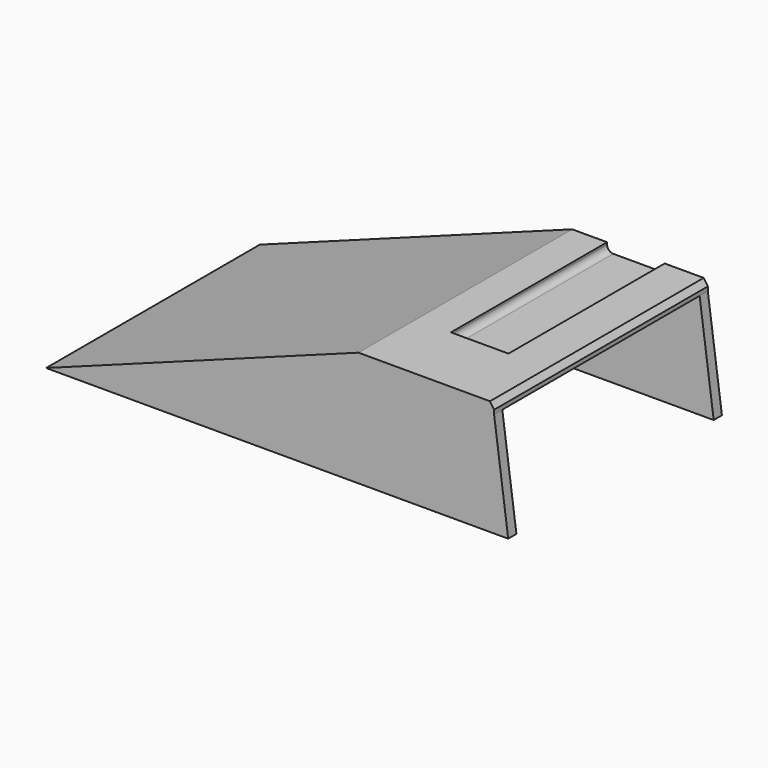
from build123d import *

# Parameters (mm, degrees)
F1_DEPTH      = 6.5
F2_R          = 6
F4_DEPTH      = 0.5
F6_DEPTH      = 3
F6_DEPTH_BACK = 25
F7_SIZE2      = 0.3
F7_SIZE       = 0.2
F8_R          = 0.3


# Not quite as in the source:
# - a pattern or mirror of a feature is missing from the dataset's text; its kind, count and spacing are read off the source's solid


with BuildPart() as f1:
    # F0 (on Front) → F1 (new body, symmetric)
    with BuildSketch(Plane.XZ):
        Polygon((15.2, 5.6), (0, 0), (7, 0), (18.8267862505, 4.7), (21.8, 5.1), (21.8, 5.6), align=None)
    extrude(amount=F1_DEPTH, both=True)

    # F2
    f2_edges = [f1.edges().sort_by_distance(p)[0] for p in [
        (18.826786, 0, 4.7),
    ]]
    fillet(f2_edges, radius=F2_R)

    # F3 (on face) → F4 (join)
    with BuildSketch(Plane(origin=(0, 6.5, 0), x_dir=(-1, 0, 0), z_dir=(0, 1, 0))):
        Polygon((-21.8, 5.6), (-21.8, 5.1), (-22.4861262499, 0), (0, 0), (-15.2, 5.6), align=None)
    f4 = extrude(amount=-F4_DEPTH)

    # F4_copies: F4 across plane
    add(f4.mirror(Plane(origin=(0, 0, 0), x_dir=(0, 0, -1), z_dir=(0, -1, 0))))

    # F5 (on Front) → F6 (cut, two sides)
    with BuildSketch(Plane.XZ) as f6_sk:
        Polygon((18.3, 5.6), (16.9, 5.6), (16.9, 5.2), (19.7, 5.2), (19.7, 5.6), align=None)
    extrude(amount=F6_DEPTH, mode=Mode.SUBTRACT)
    extrude(f6_sk.sketch, amount=-F6_DEPTH_BACK, mode=Mode.SUBTRACT)

    # F7
    f7_edges = [f1.edges().sort_by_distance(p)[0] for p in [
        (21.8, 0, 5.6),
    ]]
    f7_side = f1.faces().sort_by_distance((21.654206, 0, 5.6))[0]
    chamfer(f7_edges, length=F7_SIZE, length2=F7_SIZE2, reference=f7_side)

    # F8
    f8_edges = [f1.edges().sort_by_distance(p)[0] for p in [
        (16.9, 1.75, 5.2),
        (19.7, 1.75, 5.2),
    ]]
    fillet(f8_edges, radius=F8_R)


solid = f1.part
